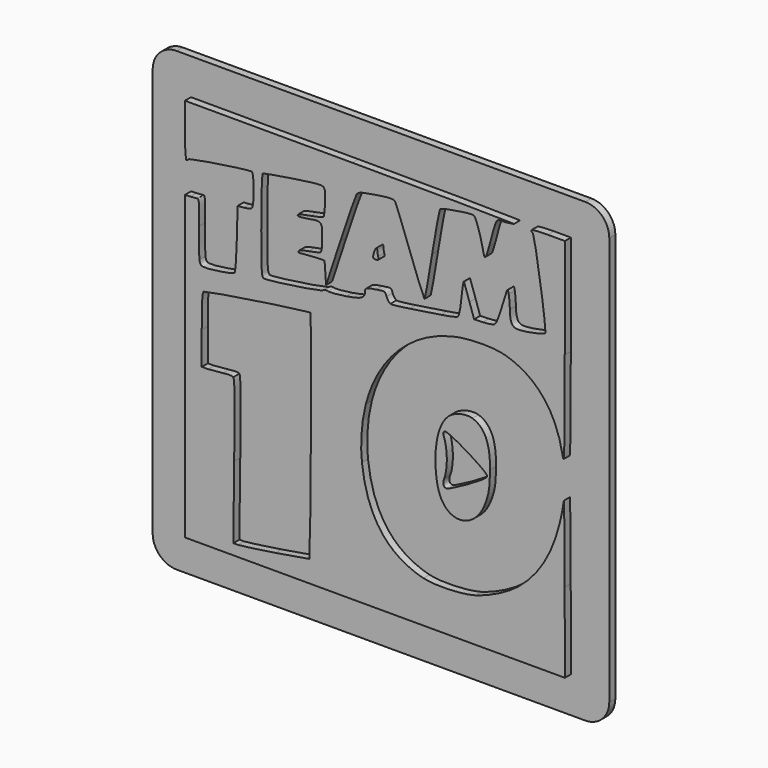
from build123d import *

# Parameters (mm, degrees)
F1_DEPTH = 2
F2_W     = 120.65
F2_H     = 120.65
F3_DEPTH = 2
F4_R     = 6.35


# Not quite as in the source:
# - ends of sketch curves that miss each other by under 0.0002 mm in the source are joined


with BuildPart() as f1:
    # F0 (on Front) → F1 (new body)
    with BuildSketch(Plane.XZ):
        with BuildLine():
            add(Edge.make_bspline(
                [(-48.8256564681, 28.949397682), (-48.0723773318, 28.9777005418), (-47.2105909978, 29.0524695479), (-46.9105769206, 29.1155179983)],
                knots=[0, 0, 0, 0, 1, 1, 1, 1], degree=3))
            Line((-48.8256564681, 28.949397682), (-50.1952530895, 28.8979085173))
            Line((-50.1952530895, 28.8979085173), (-50.1952530895, -10.9510607932))
            Line((-50.1952530895, -10.9510607932), (-50.1952530895, -50.8000080635))
            Line((-50.1952530895, -50.8000080635), (-1.02138e-05, -50.8000080635))
            Line((-1.02138e-05, -50.8000080635), (50.1952530895, -50.8000080635))
            Line((50.1952530895, -50.8000080635), (50.1403648938, -29.7341330413))
            add(Edge.make_bspline(
                [(49.9340765567, -9.6761946231), (50.0173358831, -9.121829491), (50.1101671131, -18.1479012416), (50.1403648938, -29.7341330413)],
                knots=[0, 0, 0, 0, 1, 1, 1, 1], degree=3))
            add(Edge.make_bspline(
                [(37.8886734582, -33.5827333444), (44.485489515, -28.235101233), (48.27686751, -20.7103421841), (49.9340765567, -9.6761946231)],
                knots=[0, 0, 0, 0, 1, 1, 1, 1], degree=3))
            add(Edge.make_bspline(
                [(26.6095526845, -39.3060392863), (30.1475311167, -38.3463261325), (35.133051655, -35.8165503995), (37.8886734582, -33.5827333444)],
                knots=[0, 0, 0, 0, 1, 1, 1, 1], degree=3))
            add(Edge.make_bspline(
                [(12.8110333555, -39.7741653626), (15.8573284859, -40.5562510583), (22.8788121557, -40.3180398906), (26.6095526845, -39.3060392863)],
                knots=[0, 0, 0, 0, 1, 1, 1, 1], degree=3))
            add(Edge.make_bspline(
                [(-3.4239665568, -18.1700478934), (-2.1066014789, -30.1420285892), (3.2960032261, -37.3313420358), (12.8110333555, -39.7741653626)],
                knots=[0, 0, 0, 0, 1, 1, 1, 1], degree=3))
            add(Edge.make_bspline(
                [(-2.4112483016, -4.2581322024), (-3.5386579159, -8.5678309789), (-3.9136829039, -13.7196003119), (-3.4239665568, -18.1700478934)],
                knots=[0, 0, 0, 0, 1, 1, 1, 1], degree=3))
            add(Edge.make_bspline(
                [(20.4220029693, 18.9431395692), (9.1991368846, 16.252674551), (0.6933899623, 7.6098315861), (-2.4112483016, -4.2581322024)],
                knots=[0, 0, 0, 0, 1, 1, 1, 1], degree=3))
            add(Edge.make_bspline(
                [(34.4990756581, 19.1058323635), (31.3456210086, 20.0414636272), (24.6822526449, 19.9644492072), (20.4220029693, 18.9431395692)],
                knots=[0, 0, 0, 0, 1, 1, 1, 1], degree=3))
            add(Edge.make_bspline(
                [(49.5655507438, 0.8620207128), (47.8327061343, 10.4362272035), (42.6767432475, 16.6795236076), (34.4990756581, 19.1058323635)],
                knots=[0, 0, 0, 0, 1, 1, 1, 1], degree=3))
            add(Edge.make_bspline(
                [(50.1590883241, 24.2912753801), (50.1265521306, 0.444464563), (50.066942491, -1.9082282664), (49.5655507438, 0.8620207128)],
                knots=[0, 0, 0, 0, 1, 1, 1, 1], degree=3))
            Line((50.1590883241, 24.2912753801), (50.1952530895, 50.8000080635))
            Line((50.1952530895, 50.8000080635), (45.7603320322, 50.8000080635))
            add(Edge.make_bspline(
                [(41.3254109749, 50.4304339965), (41.3254109749, 50.6336985238), (43.3211254507, 50.8000080635), (45.7603320322, 50.8000080635)],
                knots=[0, 0, 0, 0, 1, 1, 1, 1], degree=3))
            add(Edge.make_bspline(
                [(41.6619811657, 49.9264656946), (41.4768675608, 50.0003794328), (41.3254109749, 50.2271651687), (41.3254109749, 50.4304339965)],
                knots=[0, 0, 0, 0, 1, 1, 1, 1], degree=3))
            add(Edge.make_bspline(
                [(44.9781614011, 27.6465995727), (45.4579230976, 28.2246751367), (42.2635381584, 49.6862623066), (41.6619811657, 49.9264656946)],
                knots=[0, 0, 0, 0, 1, 1, 1, 1], degree=3))
            add(Edge.make_bspline(
                [(37.7099907576, 26.2063549276), (39.9379015729, 26.2063549276), (44.5396525339, 27.1182268409), (44.9781614011, 27.6465995727)],
                knots=[0, 0, 0, 0, 1, 1, 1, 1], degree=3))
            add(Edge.make_bspline(
                [(35.6577313071, 30.1635543521), (35.6936138502, 27.2448521694), (36.2322148539, 26.2063549276), (37.7099907576, 26.2063549276)],
                knots=[0, 0, 0, 0, 1, 1, 1, 1], degree=3))
            add(Edge.make_bspline(
                [(35.3537817078, 33.632662492), (35.508173405, 32.7635104262), (35.6449506709, 31.202414451), (35.6577313071, 30.1635543521)],
                knots=[0, 0, 0, 0, 1, 1, 1, 1], degree=3))
            add(Edge.make_bspline(
                [(33.6754059924, 30.4746600325), (35.0255373421, 35.0518006758), (35.0826145073, 35.1591945739), (35.3537817078, 33.632662492)],
                knots=[0, 0, 0, 0, 1, 1, 1, 1], degree=3))
            add(Edge.make_bspline(
                [(31.5426927734, 25.3429967501), (32.0334412476, 25.6056365381), (32.7422824749, 27.3112265418), (33.6754059924, 30.4746600325)],
                knots=[0, 0, 0, 0, 1, 1, 1, 1], degree=3))
            add(Edge.make_bspline(
                [(28.5070016737, 24.8724274355), (29.7723529222, 24.9148736617), (31.1384134333, 25.1266328099), (31.5426927734, 25.3429967501)],
                knots=[0, 0, 0, 0, 1, 1, 1, 1], degree=3))
            Line((28.5070016737, 24.8724274355), (26.206361916, 24.7952436821))
            Line((26.206361916, 24.7952436821), (24.9869161321, 28.4238154562))
            add(Edge.make_bspline(
                [(23.5435385512, 32.6531615268), (23.6667003407, 32.3227357175), (24.3162227518, 30.419529932), (24.9869161321, 28.4238154562)],
                knots=[0, 0, 0, 0, 1, 1, 1, 1], degree=3))
            add(Edge.make_bspline(
                [(22.8727570101, 28.835766941), (23.1185199076, 31.2657612507), (23.4203729988, 32.9835916365), (23.5435385512, 32.6531615268)],
                knots=[0, 0, 0, 0, 1, 1, 1, 1], degree=3))
            add(Edge.make_bspline(
                [(21.7978246072, 23.9583337611), (22.2442319344, 24.2847557774), (22.555160218, 25.6955686737), (22.8727570101, 28.835766941)],
                knots=[0, 0, 0, 0, 1, 1, 1, 1], degree=3))
            add(Edge.make_bspline(
                [(17.4388455254, 23.0017169885), (19.4908394182, 23.2752591564), (21.4523808113, 23.7057367847), (21.7978246072, 23.9583337611)],
                knots=[0, 0, 0, 0, 1, 1, 1, 1], degree=3))
            add(Edge.make_bspline(
                [(9.1826959603, 21.7433648517), (11.6715854841, 22.1619122736), (15.3868521702, 22.7281710577), (17.4388455254, 23.0017169885)],
                knots=[0, 0, 0, 0, 1, 1, 1, 1], degree=3))
            add(Edge.make_bspline(
                [(4.0703931242, 21.2076344515), (4.3932715041, 21.0837345836), (6.6938101994, 21.3248131293), (9.1826959603, 21.7433648517)],
                knots=[0, 0, 0, 0, 1, 1, 1, 1], degree=3))
            add(Edge.make_bspline(
                [(3.0920533019, 22.5553542793), (3.3072598621, 21.9380095052), (3.7475147442, 21.3315380824), (4.0703931242, 21.2076344515)],
                knots=[0, 0, 0, 0, 1, 1, 1, 1], degree=3))
            add(Edge.make_bspline(
                [(0.3795308679, 23.3137945886), (2.6864273585, 23.675555131), (2.7031832966, 23.6708702417), (3.0920533019, 22.5553542793)],
                knots=[0, 0, 0, 0, 1, 1, 1, 1], degree=3))
            add(Edge.make_bspline(
                [(-2.6206249565, 21.8247013039), (-2.6206249565, 22.7545913608), (-2.3592747898, 22.8843087699), (0.3795308679, 23.3137945886)],
                knots=[0, 0, 0, 0, 1, 1, 1, 1], degree=3))
            add(Edge.make_bspline(
                [(-7.61485783, 19.1592089231), (-3.5736733647, 19.8002926201), (-2.6206249565, 20.3089458114), (-2.6206249565, 21.8247013039)],
                knots=[0, 0, 0, 0, 1, 1, 1, 1], degree=3))
            add(Edge.make_bspline(
                [(-12.3715084883, 18.7713307274), (-11.9478122575, 18.6368558575), (-9.8073177679, 18.8114062868), (-7.61485783, 19.1592089231)],
                knots=[0, 0, 0, 0, 1, 1, 1, 1], degree=3))
            add(Edge.make_bspline(
                [(-13.660336865, 18.5855354886), (-13.375175204, 18.8221990032), (-12.7952004186, 18.9058055974), (-12.3715084883, 18.7713307274)],
                knots=[0, 0, 0, 0, 1, 1, 1, 1], degree=3))
            add(Edge.make_bspline(
                [(-29.3748302516, 16.2509527265), (-28.5107103428, 15.9193539479), (-14.3354124849, 18.0252721802), (-13.660336865, 18.5855354886)],
                knots=[0, 0, 0, 0, 1, 1, 1, 1], degree=3))
            add(Edge.make_bspline(
                [(-30.0365005834, 28.3873684686), (-30.0365005834, 17.7428725342), (-29.9675614826, 16.4784039694), (-29.3748302516, 16.2509527265)],
                knots=[0, 0, 0, 0, 1, 1, 1, 1], degree=3))
            add(Edge.make_bspline(
                [(-29.5958065097, 40.5422453088), (-29.8984858401, 40.3551760381), (-30.0365005834, 36.5485827697), (-30.0365005834, 28.3873684686)],
                knots=[0, 0, 0, 0, 1, 1, 1, 1], degree=3))
            add(Edge.make_bspline(
                [(-21.6524032769, 41.9588800469), (-25.7788914329, 41.3295324949), (-29.3534222157, 40.6920445781), (-29.5958065097, 40.5422453088)],
                knots=[0, 0, 0, 0, 1, 1, 1, 1], degree=3))
            add(Edge.make_bspline(
                [(-13.5874509533, 42.6365279209), (-14.0183075658, 42.994111574), (-15.9029313008, 42.8357564013), (-21.6524032769, 41.9588800469)],
                knots=[0, 0, 0, 0, 1, 1, 1, 1], degree=3))
            add(Edge.make_bspline(
                [(-13.166512437, 39.058292232), (-13.0617714281, 41.3647296411), (-13.1707054533, 42.2906524594), (-13.5874509533, 42.6365279209)],
                knots=[0, 0, 0, 0, 1, 1, 1, 1], degree=3))
            add(Edge.make_bspline(
                [(-13.5977157797, 35.6567765895), (-13.438272573, 35.8162240968), (-13.2442321439, 37.346904577), (-13.166512437, 39.058292232)],
                knots=[0, 0, 0, 0, 1, 1, 1, 1], degree=3))
            add(Edge.make_bspline(
                [(-16.9785528636, 34.8293815901), (-15.2785384964, 35.1250053643), (-13.7571632869, 35.4973328452), (-13.5977157797, 35.6567765895)],
                knots=[0, 0, 0, 0, 1, 1, 1, 1], degree=3))
            add(Edge.make_bspline(
                [(-20.2820970681, 34.0792789324), (-20.1651645956, 34.1962119425), (-18.6785709937, 34.5337578159), (-16.9785528636, 34.8293815901)],
                knots=[0, 0, 0, 0, 1, 1, 1, 1], degree=3))
            add(Edge.make_bspline(
                [(-17.6122466382, 33.9168361064), (-19.9270657793, 33.5090894644), (-20.7992212274, 33.5621553107), (-20.2820970681, 34.0792789324)],
                knots=[0, 0, 0, 0, 1, 1, 1, 1], degree=3))
            add(Edge.make_bspline(
                [(-13.9095149205, 30.6777229725), (-13.9095149205, 34.466649128), (-14.0069622314, 34.5518963743), (-17.6122466382, 33.9168361064)],
                knots=[0, 0, 0, 0, 1, 1, 1, 1], degree=3))
            add(Edge.make_bspline(
                [(-14.4073065869, 27.1558150815), (-14.0797191272, 27.3582770225), (-13.9095149205, 28.5624871054), (-13.9095149205, 30.6777229725)],
                knots=[0, 0, 0, 0, 1, 1, 1, 1], degree=3))
            add(Edge.make_bspline(
                [(-17.4996034063, 26.4226016783), (-16.0726275074, 26.6566606848), (-14.6810944225, 26.9866064474), (-14.4073065869, 27.1558150815)],
                knots=[0, 0, 0, 0, 1, 1, 1, 1], degree=3))
            add(Edge.make_bspline(
                [(-20.2489889041, 25.5323759428), (-20.1638018653, 25.7879402846), (-18.9265798427, 26.1885383714), (-17.4996034063, 26.4226016783)],
                knots=[0, 0, 0, 0, 1, 1, 1, 1], degree=3))
            add(Edge.make_bspline(
                [(-18.6686007536, 25.3293167658), (-19.8960777763, 25.1442676688), (-20.3585513442, 25.203691848), (-20.2489889041, 25.5323759428)],
                knots=[0, 0, 0, 0, 1, 1, 1, 1], degree=3))
            add(Edge.make_bspline(
                [(-15.1190388452, 25.596254933), (-16.1168960831, 25.5934327105), (-17.7141976786, 25.4731936683), (-18.6686007536, 25.3293167658)],
                knots=[0, 0, 0, 0, 1, 1, 1, 1], degree=3))
            Line((-15.1190388452, 25.596254933), (-13.3047529581, 25.6015768382))
            Line((-13.3047529581, 25.6015768382), (-13.1031656373, 22.825755448))
            Line((-13.1031656373, 22.825755448), (-12.9015783166, 20.0499345952))
            Line((-12.9015783166, 20.0499345952), (-9.13506007, 31.4940102418))
            add(Edge.make_bspline(
                [(-4.8412383108, 43.7695292987), (-5.1312541945, 43.3122362562), (-7.0634724272, 37.7882517936), (-9.13506007, 31.4940102418)],
                knots=[0, 0, 0, 0, 1, 1, 1, 1], degree=3))
            add(Edge.make_bspline(
                [(0.2379117433, 45.2912071579), (-3.4702993866, 44.7288994853), (-4.4116637937, 44.44687076), (-4.8412383108, 43.7695292987)],
                knots=[0, 0, 0, 0, 1, 1, 1, 1], degree=3))
            add(Edge.make_bspline(
                [(5.2596373644, 45.467700889), (4.8796812817, 45.8831277391), (3.9186543161, 45.8493497677), (0.2379117433, 45.2912071579)],
                knots=[0, 0, 0, 0, 1, 1, 1, 1], degree=3))
            add(Edge.make_bspline(
                [(9.2975561151, 34.9775482709), (7.3351358012, 40.4645734453), (5.5180680091, 45.1851437362), (5.2596373644, 45.467700889)],
                knots=[0, 0, 0, 0, 1, 1, 1, 1], degree=3))
            add(Edge.make_bspline(
                [(13.1329322899, 25.3013568731), (12.9859025616, 25.1362326669), (11.2599807295, 29.4905187959), (9.2975561151, 34.9775482709)],
                knots=[0, 0, 0, 0, 1, 1, 1, 1], degree=3))
            add(Edge.make_bspline(
                [(15.1188093044, 36.3809508172), (14.1736109753, 30.4522956664), (13.2799663187, 25.4664767788), (13.1329322899, 25.3013568731)],
                knots=[0, 0, 0, 0, 1, 1, 1, 1], degree=3))
            add(Edge.make_bspline(
                [(17.299274528, 47.5436831354), (17.0452180593, 47.3328351619), (16.0640081712, 42.3096016676), (15.1188093044, 36.3809508172)],
                knots=[0, 0, 0, 0, 1, 1, 1, 1], degree=3))
            add(Edge.make_bspline(
                [(26.14556318, 48.9532461903), (25.3883888391, 49.243802328), (17.9124709038, 48.0525905955), (17.299274528, 47.5436831354)],
                knots=[0, 0, 0, 0, 1, 1, 1, 1], degree=3))
            add(Edge.make_bspline(
                [(28.6720812619, 41.1993957841), (27.9435651121, 44.8600038152), (26.6761651988, 48.7496349328), (26.14556318, 48.9532461903)],
                knots=[0, 0, 0, 0, 1, 1, 1, 1], degree=3))
            add(Edge.make_bspline(
                [(30.2117933916, 43.1396737466), (29.3498984693, 39.9052895825), (29.0138970235, 39.481871811), (28.6720812619, 41.1993957841)],
                knots=[0, 0, 0, 0, 1, 1, 1, 1], degree=3))
            add(Edge.make_bspline(
                [(33.5929083972, 50.0168773392), (31.9501007487, 49.991154797), (32.1410646865, 50.3795614203), (30.2117933916, 43.1396737466)],
                knots=[0, 0, 0, 0, 1, 1, 1, 1], degree=3))
            add(Edge.make_bspline(
                [(36.6889025968, 50.373686897), (35.8019183854, 50.1902182446), (34.4087199204, 50.0296542123), (33.5929083972, 50.0168773392)],
                knots=[0, 0, 0, 0, 1, 1, 1, 1], degree=3))
            add(Edge.make_bspline(
                [(-5.9468157494, 50.7536268527), (18.565267093, 50.7279446281), (37.5822811581, 50.5584741992), (36.6889025968, 50.373686897)],
                knots=[0, 0, 0, 0, 1, 1, 1, 1], degree=3))
            Line((-5.9468157494, 50.7536268527), (-50.195232662, 50.7999919365))
            Line((-50.195232662, 50.7999919365), (-50.195232662, 43.9460230298))
            add(Edge.make_bspline(
                [(-49.8256542945, 37.0920541231), (-50.0351481388, 37.0920541231), (-50.195232662, 40.0608827402), (-50.195232662, 43.9460230298)],
                knots=[0, 0, 0, 0, 1, 1, 1, 1], degree=3))
            add(Edge.make_bspline(
                [(-49.3216859925, 37.4410942367), (-49.3956040313, 37.2491228999), (-49.6223897672, 37.0920541231), (-49.8256542945, 37.0920541231)],
                knots=[0, 0, 0, 0, 1, 1, 1, 1], degree=3))
            add(Edge.make_bspline(
                [(-32.5563942371, 40.0214162433), (-33.2842937985, 40.300739398), (-49.1615127709, 37.8570978954), (-49.3216859925, 37.4410942367)],
                knots=[0, 0, 0, 0, 1, 1, 1, 1], degree=3))
            add(Edge.make_bspline(
                [(-32.5614747752, 31.5270184184), (-31.8519234229, 32.1158909994), (-31.847375613, 39.7493335677), (-32.5563942371, 40.0214162433)],
                knots=[0, 0, 0, 0, 1, 1, 1, 1], degree=3))
            add(Edge.make_bspline(
                [(-34.6781416434, 30.9736811128), (-33.7939672904, 31.0456397229), (-32.8414671997, 31.2946403815), (-32.5614747752, 31.5270184184)],
                knots=[0, 0, 0, 0, 1, 1, 1, 1], degree=3))
            Line((-34.6781416434, 30.9736811128), (-36.2857279553, 30.8428471787))
            Line((-36.2857279553, 30.8428471787), (-36.487315276, 23.100821616))
            add(Edge.make_bspline(
                [(-37.0920772384, 14.9934069391), (-36.8642830283, 15.1998484825), (-36.6012121123, 18.7266105962), (-36.487315276, 23.100821616)],
                knots=[0, 0, 0, 0, 1, 1, 1, 1], degree=3))
            add(Edge.make_bspline(
                [(-44.7109931555, 13.7079249119), (-42.6529236897, 13.7079249119), (-37.5628798568, 14.5667309788), (-37.0920772384, 14.9934069391)],
                knots=[0, 0, 0, 0, 1, 1, 1, 1], degree=3))
            add(Edge.make_bspline(
                [(-46.366190092, 15.018242497), (-46.1500003233, 13.8340701937), (-45.9906490404, 13.7079249119), (-44.7109931555, 13.7079249119)],
                knots=[0, 0, 0, 0, 1, 1, 1, 1], degree=3))
            add(Edge.make_bspline(
                [(-46.4852561647, 22.7793543472), (-46.551344552, 19.2314175014), (-46.4977545786, 15.7389171688), (-46.366190092, 15.018242497)],
                knots=[0, 0, 0, 0, 1, 1, 1, 1], degree=3))
            add(Edge.make_bspline(
                [(-46.9105769206, 29.1155179983), (-46.4661010687, 29.2089211987), (-46.3873449342, 28.0356389113), (-46.4852561647, 22.7793543472)],
                knots=[0, 0, 0, 0, 1, 1, 1, 1], degree=3))
        make_face()
        with BuildLine():
            add(Edge.make_bspline(
                [(-26.2947619879, -46.6123174594), (-21.4649716866, -45.8713953571), (-17.4446308127, -45.1951666577), (-17.3606737254, -45.1095888083)],
                knots=[0, 0, 0, 0, 1, 1, 1, 1], degree=3))
            add(Edge.make_bspline(
                [(-36.248865429, -47.9686087801), (-35.6038988914, -47.9635690971), (-31.1245560521, -47.3532271977), (-26.2947619879, -46.6123174594)],
                knots=[0, 0, 0, 0, 1, 1, 1, 1], degree=3))
            Line((-36.248865429, -47.9686087801), (-37.421527365, -47.9778011619))
            Line((-37.421527365, -47.9778011619), (-37.1828920576, -28.8540587057))
            add(Edge.make_bspline(
                [(-37.4213419047, -9.3500220376), (-37.0599802364, -9.638074192), (-37.0021408023, -14.3688770552), (-37.1828920576, -28.8540587057)],
                knots=[0, 0, 0, 0, 1, 1, 1, 1], degree=3))
            add(Edge.make_bspline(
                [(-40.1158870502, -9.2935329698), (-38.8025859727, -9.1017589197), (-37.7038985199, -9.1247882553), (-37.4213419047, -9.3500220376)],
                knots=[0, 0, 0, 0, 1, 1, 1, 1], degree=3))
            add(Edge.make_bspline(
                [(-44.0468398055, -9.6467784637), (-43.1044190808, -9.6306111606), (-41.3354898034, -9.4716313359), (-40.1158870502, -9.2935329698)],
                knots=[0, 0, 0, 0, 1, 1, 1, 1], degree=3))
            Line((-44.0468398055, -9.6467784637), (-45.7603320322, -9.6762102125))
            Line((-45.7603320322, -9.6762102125), (-45.7603320322, -1.0573206594))
            add(Edge.make_bspline(
                [(-45.2563637302, 7.9546308401), (-45.6315618146, 7.6619986218), (-45.7603320322, 5.3593714818), (-45.7603320322, -1.0573206594)],
                knots=[0, 0, 0, 0, 1, 1, 1, 1], degree=3))
            add(Edge.make_bspline(
                [(-17.0229101376, 12.2275762164), (-17.557350379, 12.5578773103), (-44.6022284637, 8.4648160951), (-45.2563637302, 7.9546308401)],
                knots=[0, 0, 0, 0, 1, 1, 1, 1], degree=3))
            add(Edge.make_bspline(
                [(-17.3606737254, -45.1095888083), (-16.9754403553, -44.7169128344), (-16.6413822113, 11.991779796), (-17.0229101376, 12.2275762164)],
                knots=[0, 0, 0, 0, 1, 1, 1, 1], degree=3))
        make_face(mode=Mode.SUBTRACT)
    extrude(amount=F1_DEPTH)



with BuildPart() as f1b:
    # F0 (on Front) → F1, piece 2 (new body)
    with BuildSketch(Plane.XZ):
        with BuildLine():
            add(Edge.make_bspline(
                [(19.3074755912, -21.9830919561), (17.2546151417, -20.3646844368), (16.2266203306, -17.4030280278), (16.013598977, -12.4933930205)],
                knots=[0, 0, 0, 0, 1, 1, 1, 1], degree=3))
            add(Edge.make_bspline(
                [(28.5681143483, -18.4286118546), (26.5675295228, -22.657498306), (22.2600761602, -24.3108169862), (19.3074755912, -21.9830919561)],
                knots=[0, 0, 0, 0, 1, 1, 1, 1], degree=3))
            add(Edge.make_bspline(
                [(30.4298178737, -8.8331440836), (30.4184483488, -13.2938559539), (30.0160316756, -15.367959944), (28.5681143483, -18.4286118546)],
                knots=[0, 0, 0, 0, 1, 1, 1, 1], degree=3))
            add(Edge.make_bspline(
                [(25.7629058272, 1.6259683877), (28.9950886577, 0.559248921), (30.4454734139, -2.6912380383), (30.4298178737, -8.8331440836)],
                knots=[0, 0, 0, 0, 1, 1, 1, 1], degree=3))
            add(Edge.make_bspline(
                [(20.1347894181, 0.5519874769), (21.7635547627, 1.6191950537), (24.3106750687, 2.1052462746), (25.7629058272, 1.6259683877)],
                knots=[0, 0, 0, 0, 1, 1, 1, 1], degree=3))
            add(Edge.make_bspline(
                [(16.013598977, -12.4933930205), (15.7410975372, -6.2128475801), (17.289162908, -1.312542034), (20.1347894181, 0.5519874769)],
                knots=[0, 0, 0, 0, 1, 1, 1, 1], degree=3))
        make_face()
        with BuildLine():
            add(Edge.make_bspline(
                [(24.6072782885, -14.0876261882), (28.1670485789, -12.0720959476), (29.6333264794, -11.0270350227), (29.6333264794, -10.5054114344)],
                knots=[0, 0, 0, 0, 1, 1, 1, 1], degree=3))
            add(Edge.make_bspline(
                [(18.9501816863, -16.9333537608), (19.2972591458, -16.9333537608), (21.8429522136, -15.6527743373), (24.6072782885, -14.0876261882)],
                knots=[0, 0, 0, 0, 1, 1, 1, 1], degree=3))
            add(Edge.make_bspline(
                [(18.3037072755, -14.823021035), (17.8278246566, -16.0746885362), (18.0908633187, -16.9333537608), (18.9501816863, -16.9333537608)],
                knots=[0, 0, 0, 0, 1, 1, 1, 1], degree=3))
            add(Edge.make_bspline(
                [(18.1146753506, -4.7084938664), (19.2199780929, -7.5888665048), (19.3059150365, -12.1870168474), (18.3037072755, -14.823021035)],
                knots=[0, 0, 0, 0, 1, 1, 1, 1], degree=3))
            add(Edge.make_bspline(
                [(18.5074884039, -3.7891750487), (18.0998385238, -3.9456068096), (17.9534210834, -4.288273001), (18.1146753506, -4.7084938664)],
                knots=[0, 0, 0, 0, 1, 1, 1, 1], degree=3))
            add(Edge.make_bspline(
                [(29.6333264794, -10.5054114344), (29.6333264794, -9.551984042), (19.4730830694, -3.4186414261), (18.5074884039, -3.7891750487)],
                knots=[0, 0, 0, 0, 1, 1, 1, 1], degree=3))
        make_face(mode=Mode.SUBTRACT)
    extrude(amount=F1_DEPTH)


with BuildPart() as f1c:
    # F0 (on Front) → F1, piece 3 (new body)
    with BuildSketch(Plane.XZ):
        with BuildLine():
            add(Edge.make_bspline(
                [(-0.3588109167, 31.3468154806), (-0.0539786337, 32.6401594133), (0.6020026351, 33.5134921314), (0.6102553512, 32.6369743337)],
                knots=[0, 0, 0, 0, 1, 1, 1, 1], degree=3))
            add(Edge.make_bspline(
                [(0.2409194261, 30.2380852163), (-0.4929793739, 30.2380852163), (-0.5815450162, 30.4018144383), (-0.3588109167, 31.3468154806)],
                knots=[0, 0, 0, 0, 1, 1, 1, 1], degree=3))
            add(Edge.make_bspline(
                [(0.8588689622, 31.1452281599), (1.0554246635, 30.4117685514), (0.9371133337, 30.2380852163), (0.2409194261, 30.2380852163)],
                knots=[0, 0, 0, 0, 1, 1, 1, 1], degree=3))
            add(Edge.make_bspline(
                [(0.6102553512, 32.6369743337), (0.6134807484, 32.315442557), (0.7251601241, 31.6441567788), (0.8588689622, 31.1452281599)],
                knots=[0, 0, 0, 0, 1, 1, 1, 1], degree=3))
        make_face()
    extrude(amount=F1_DEPTH)


with BuildPart() as f1_1:
    add(f1.part)

    add(f1b.part)  # F3 merges F1b

    add(f1c.part)  # F3 merges F1c
    # F2 (on Front) → F3 (join)
    with BuildSketch(Plane.XZ):
        Rectangle(F2_W, F2_H)
    extrude(amount=-F3_DEPTH)

    # F4
    f4_edges = [f1_1.edges().sort_by_distance(p)[0] for p in [
        (-60.325, 1, 60.325),
        (60.325, 1, 60.325),
        (60.325, 1, -60.325),
        (-60.325, 1, -60.325),
    ]]
    fillet(f4_edges, radius=F4_R)


solid = f1_1.part
